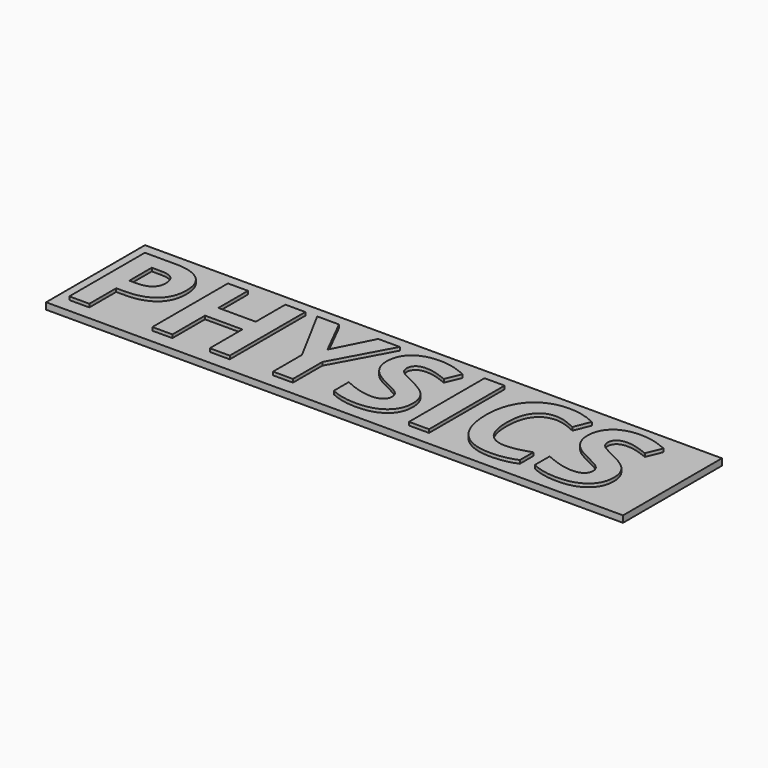
from build123d import *

# Parameters (mm, degrees)
F0_W         = 35
F0_H         = 7.5
F1_DEPTH     = 0.4
F2_TEXT_SIZE = 8.0246209962
F3_DEPTH     = 0.2


# Not quite as in the source:
# - Text() gives the source's letters only with a copy of the font that has no kerning and outlines rounded to 1/6400 em; it was checked with that copy


with BuildPart() as f1:
    # F0 (on Top) → F1 (new body)
    with BuildSketch(Plane.XY):
        Rectangle(F0_W, F0_H)
    extrude(amount=F1_DEPTH)

    # F2 (on face) → F3 (join)
    with BuildSketch(Plane.XY.offset(0.4)):
        with Locations((-17.5, -2.8888635586)):
            Text('PHYSICS', F2_TEXT_SIZE, font='Open Sans', font_style=FontStyle.BOLD, text_align=(TextAlign.LEFT, TextAlign.BOTTOM))
    extrude(amount=F3_DEPTH)


solid = f1.part
